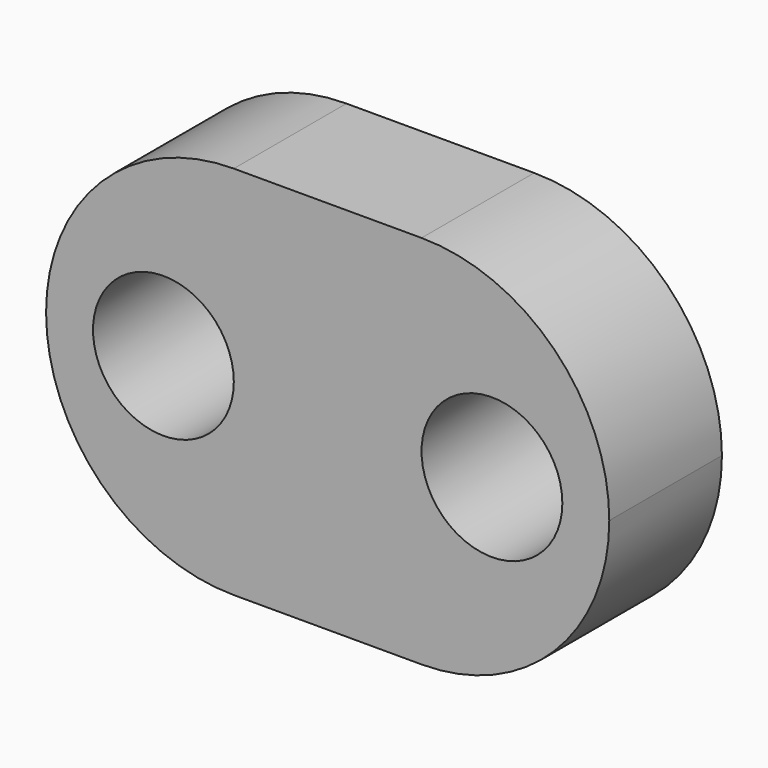
from build123d import *

# Parameters (mm, degrees)
F0_W     = 12
F0_H     = 3
F1_DEPTH = 4
F2_R     = 1.5
F3_DEPTH = 25
F4_R     = 3.99999


# Not quite as in the source:
# - a fillet or chamfer is up to 0.001 mm smaller than in the source, because OpenCascade refuses the exact size


with BuildPart() as f1:
    # F0 (on Top) → F1 (new body, symmetric)
    with BuildSketch(Plane.XY):
        Rectangle(F0_W, F0_H)
    extrude(amount=F1_DEPTH, both=True)

    # F2 (on face) → F3 (cut)
    with BuildSketch(Plane.XZ.offset(1.5)):
        with Locations((-3.5, 0)):
            Circle(F2_R)
        with Locations((3.5, 0)):
            Circle(F2_R)
    extrude(amount=-F3_DEPTH, mode=Mode.SUBTRACT)

    # F4 (radius 4 in the source; OpenCascade refuses exactly that, so slightly less here)
    f4_edges = [f1.edges().sort_by_distance(p)[0] for p in [
        (-6, 0, 4),
        (-6, 0, -4),
        (6, 0, 4),
        (6, 0, -4),
    ]]
    fillet(f4_edges, radius=F4_R)


solid = f1.part
